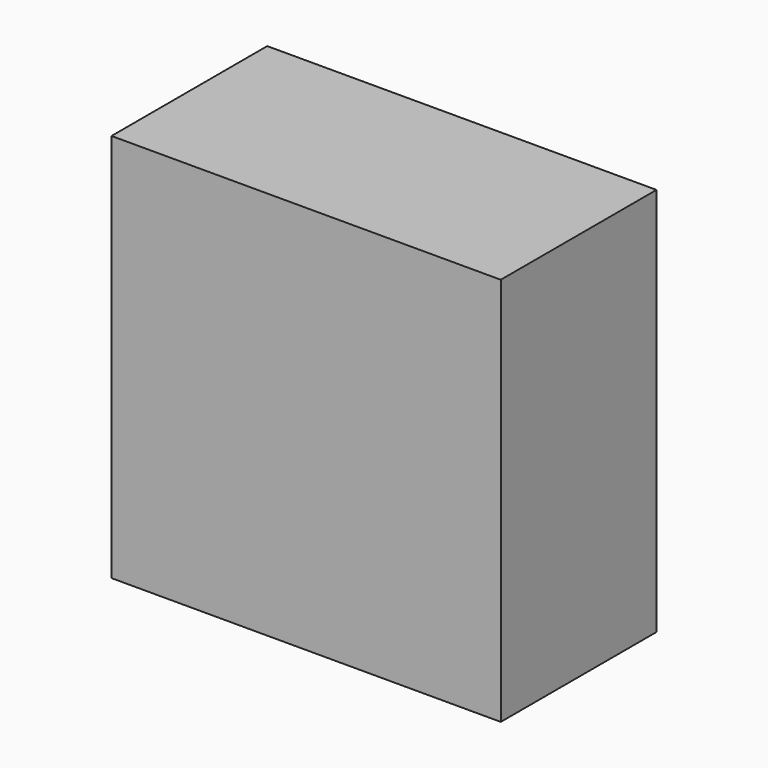
from build123d import *

# Parameters (mm, degrees)
F0_W     = 25.4
F0_H     = 25.4
F1_DEPTH = 12.7
F2_R     = 5.08
F3_DEPTH = 5.08
F4_R     = 5.07999


# Not quite as in the source:
# - a fillet or chamfer is up to 0.001 mm smaller than in the source, because OpenCascade refuses the exact size


with BuildPart() as f1:
    # F0 (on Front) → F1 (new body)
    with BuildSketch(Plane.XZ):
        with Locations((24.4342711151, -0.3571881309)):
            Rectangle(F0_W, F0_H)
    extrude(amount=F1_DEPTH)

    # F2 (on Front) → F3 (join)
    with BuildSketch(Plane.XZ):
        with Locations((24.4607284337, 0)):
            Circle(F2_R)
    extrude(amount=-F3_DEPTH)

    # F4 (radius 5.08 in the source; OpenCascade refuses exactly that, so slightly less here)
    f4_edges = [f1.edges().sort_by_distance(p)[0] for p in [
        (19.380728, 5.08, 0),
    ]]
    fillet(f4_edges, radius=F4_R)


solid = f1.part
